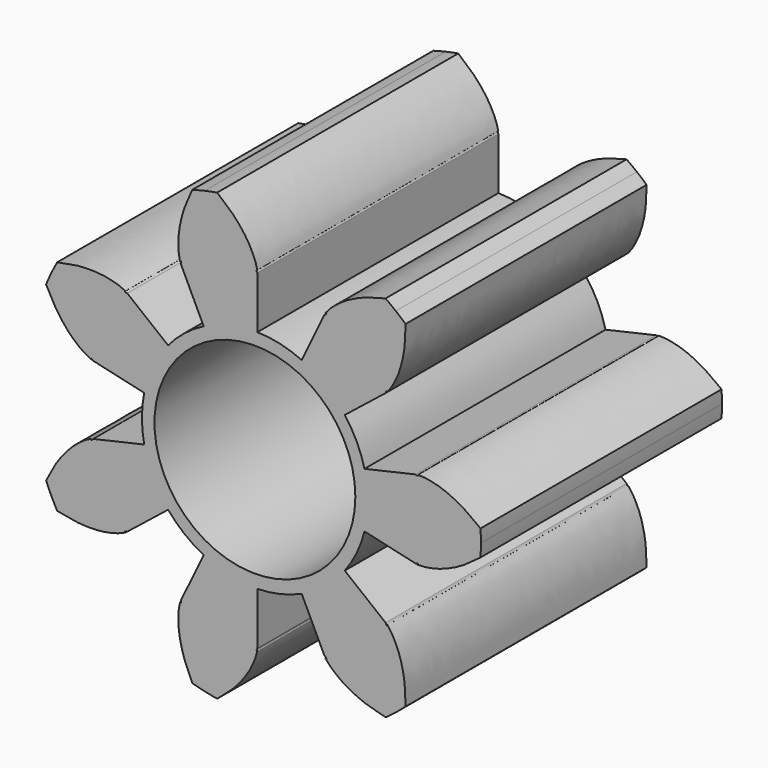
from build123d import *

# Parameters (mm, degrees)
F7_DEPTH  = 12
F8_DEPTH  = 12
F12_COUNT = 7
F13_R     = 4
F14_DEPTH = 12


with BuildPart() as f7:
    # F6 (on Front) → F7 (new body)
    with BuildSketch(Plane.XZ):
        with BuildLine():
            ThreePointArc((-39.0566174341, 53.5192313022), (-39.3688059254, 45.6716665645), (-32.5157936507, 49.5080654919))
            ThreePointArc((-32.5157936507, 49.5080654919), (-33.7994380125, 52.6554330331), (-36.9180958368, 54.0073349017))
            ThreePointArc((-36.9180958368, 54.0073349017), (-37.4712667511, 53.985328891), (-38.0175502503, 53.8955699722))
            ThreePointArc((-38.0175502503, 53.8955699722), (-38.5486796114, 53.7394164364), (-39.0566174341, 53.5192313022))
        make_face()
    extrude(amount=F7_DEPTH)

    # F5 (on Front) → F8 (join)
    with BuildSketch(Plane.XZ):
        with BuildLine():
            Line((-36.9180958368, 54.0073349017), (-36.9180958368, 56.0851832472))
            add(Edge.make_bspline(
                [(-36.9180958368, 56.0851832472), (-36.9992763265, 56.2395751396), (-36.8897351126, 56.1214509955), (-36.9517903268, 56.2762613124), (-36.9601028005, 56.3397622343), (-36.9892825172, 56.4292805319), (-37.0158024339, 56.5161441761), (-37.1873279574, 56.9168814222), (-37.4604346943, 57.3380905686), (-37.9354913593, 57.9112391709), (-38.231263722, 58.1168811972), (-38.5186673986, 58.3817560614)],
                knots=[0, 0, 0, 0, 0.06642628, 0.1307017559, 0.1946025272, 0.2576323816, 0.3229318542, 0.4626396647, 0.6235980721, 0.8033116217, 1, 1, 1, 1], degree=3))
            ThreePointArc((-38.5186673986, 58.3817560614), (-38.7694470812, 58.335629293), (-39.0188193894, 58.2824167016))
            ThreePointArc((-39.0188193894, 58.2824167016), (-39.2665841538, 58.2221610003), (-39.5125424953, 58.1549105562))
            add(Edge.make_bspline(
                [(-39.9581620436, 55.3913079737), (-39.9520090813, 55.5656331567), (-39.9994501593, 55.4116788289), (-40.0107100225, 55.5780828532), (-40.0307727598, 55.6389018541), (-40.0433232772, 55.7322156579), (-40.0571183806, 55.8219836577), (-40.0764525986, 56.2574575761), (-40.0131477305, 56.7554504761), (-39.8338163235, 57.4779588856), (-39.656559364, 57.7915667679), (-39.5125424953, 58.1549105562)],
                knots=[0, 0, 0, 0, 0.06642628, 0.1307017559, 0.1946025272, 0.2576323816, 0.3229318542, 0.4626396647, 0.6235980721, 0.8033116217, 1, 1, 1, 1], degree=3))
            Line((-39.9581620436, 55.3913079737), (-39.0566174341, 53.5192313022))
            ThreePointArc((-39.0566174341, 53.5192313022), (-38.5486796114, 53.7394164364), (-38.0175502503, 53.8955699722))
            ThreePointArc((-38.0175502503, 53.8955699722), (-37.4712667511, 53.985328891), (-36.9180958368, 54.0073349017))
        make_face()
    extrude(amount=F8_DEPTH)

    # F12: F7 ×7 about axis
    f12_axis = Axis((-37.0161309838, 15.3900273144, 49.5080654919), (0, 1, 0))


with BuildPart() as f7_1:
    add(f7.part)
    for i in range(1, F12_COUNT):
        add(f7.part.rotate(f12_axis, i * 360 / F12_COUNT))

    # F13 (on Front) → F14 (cut)
    with BuildSketch(Plane.XZ):
        with Locations((-37.0161309838, 49.5080654919)):
            Circle(F13_R)
    extrude(amount=F14_DEPTH, mode=Mode.SUBTRACT)


solid = f7_1.part
